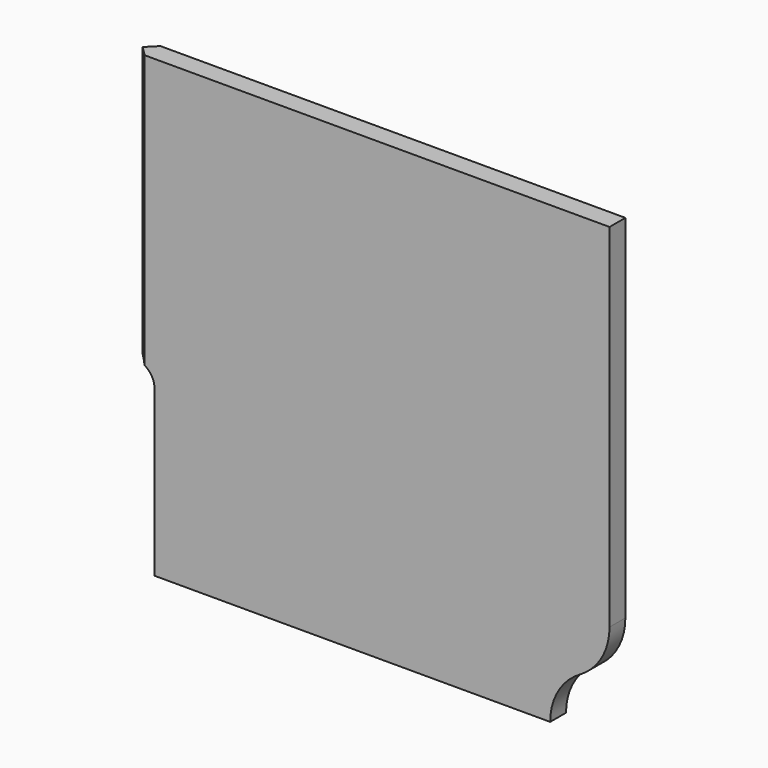
from build123d import *

# Parameters (mm, degrees)
F1_DEPTH = 19.05
F2_SIZE  = 9.52499


# Not quite as in the source:
# - a fillet or chamfer is up to 0.001 mm smaller than in the source, because OpenCascade refuses the exact size


with BuildPart() as f1:
    # F0 (on Front) → F1 (new body)
    with BuildSketch(Plane.XZ):
        with BuildLine():
            Line((301.9656721215, 276.6333943507), (-155.2343278785, 276.6333943507))
            Line((-155.2343278785, 276.6333943507), (-155.2343278785, 16.2833943507))
            ThreePointArc((-155.2343278785, 16.2833943507), (-141.7639436969, 10.7037785323), (-136.1843278785, -2.7666056493))
            Line((-136.1843278785, -2.7666056493), (-136.1843278785, -161.5166056493))
            Line((-136.1843278785, -161.5166056493), (244.8156721215, -161.5166056493))
            ThreePointArc((244.8156721215, -161.5166056493), (252.4723202952, -132.9416056493), (273.3906721215, -112.023253823))
            ThreePointArc((273.3906721215, -112.023253823), (294.3090239478, -91.1049019968), (301.9656721215, -62.5299019968))
            Line((301.9656721215, -62.5299019968), (301.9656721215, 276.6333943507))
        make_face()
    extrude(amount=-F1_DEPTH)

    # F2 (size 9.525 in the source; OpenCascade refuses exactly that, so slightly less here)
    f2_edges = [f1.edges().sort_by_distance(p)[0] for p in [
        (-155.234328, 0, 146.458394),
        (-155.234328, 19.05, 146.458394),
    ]]
    chamfer(f2_edges, length=F2_SIZE)


solid = f1.part
